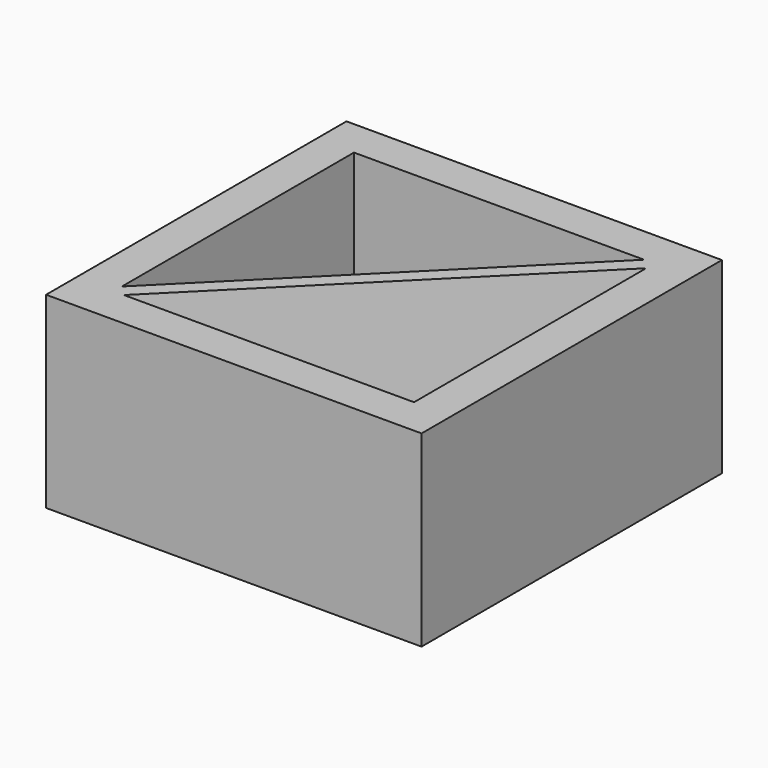
from build123d import *

# Parameters (mm, degrees)
F0_W     = 31.75
F0_H     = 31.75
F1_DEPTH = 3.175
F2_W     = 31.75
F2_H     = 31.75
F3_DEPTH = 12.7


# Not quite as in the source:
# - a length typed as a fraction of an inch, garbled in the dataset ("3 / 203.2 mm" for 3/8 in), is restored


with BuildPart() as f1:
    # F0 (on Top) → F1 (new body)
    with BuildSketch(Plane.XY):
        Rectangle(F0_W, F0_H)
    extrude(amount=F1_DEPTH)

    # F2 (on face) → F3 (join)
    with BuildSketch(Plane.XY.offset(3.175)):
        Rectangle(F2_W, F2_H)
        Polygon((12.7, 11.8309138343), (12.7, -12.7), (-11.8309138343, -12.7), (-12.7, -12.7), (-12.7, -11.8309138343), (-12.7, 12.7), (11.8309138343, 12.7), (12.7, 12.7), align=None, mode=Mode.SUBTRACT)
        Polygon((-12.7, -11.8309138343), (-12.7, -12.7), (12.7, 12.7), (11.8309138343, 12.7), align=None)
        Polygon((-12.7, -12.7), (-11.8309138343, -12.7), (12.7, 11.8309138343), (12.7, 12.7), align=None)
    extrude(amount=F3_DEPTH)


solid = f1.part
